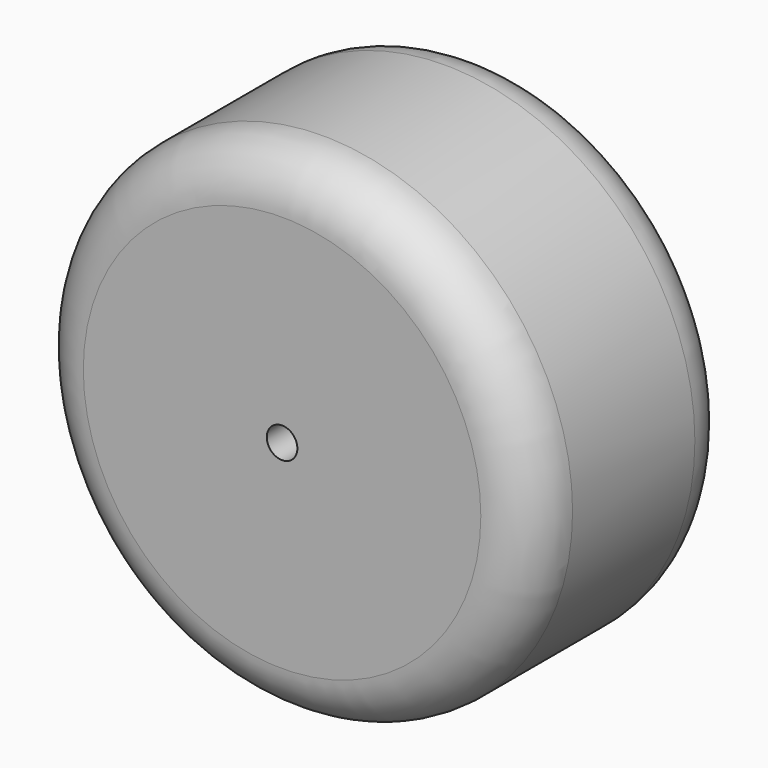
from build123d import *

# Parameters (mm, degrees)
F0_R     = 49
F1_DEPTH = 50
F2_R     = 10
F4_R     = 25.5
F4_R_2   = 6.5
F5_DEPTH = 12
F6_DEPTH = 15
F7_R     = 11.99999
F4_R_3   = 3
F8_DEPTH = 50.001


# Not quite as in the source:
# - a fillet or chamfer is up to 0.001 mm smaller than in the source, because OpenCascade refuses the exact size


with BuildPart() as f1:
    # F0 (on Front) → F1 (new body)
    with BuildSketch(Plane.XZ):
        Circle(F0_R)
    extrude(amount=F1_DEPTH)

    # F2
    f2_edges = [f1.edges().sort_by_distance(p)[0] for p in [
        (-49, -50, 0),
        (-49, 0, 0),
    ]]
    fillet(f2_edges, radius=F2_R)

    # F4 (on Front) → F5 (cut)
    with BuildSketch(Plane.XZ):
        Circle(F4_R)
        Circle(F4_R_2, mode=Mode.SUBTRACT)
    extrude(amount=F5_DEPTH, mode=Mode.SUBTRACT)

    # F6 (cut): a face of the model
    f6_faces = [f1.faces().sort_by_distance(p)[0] for p in [
        (0, 0, 0),
    ]]
    extrude(f6_faces, amount=-F6_DEPTH, mode=Mode.SUBTRACT)

    # F7 (radius 12 in the source; OpenCascade refuses exactly that, so slightly less here)
    f7_edges = [f1.edges().sort_by_distance(p)[0] for p in [
        (-25.5, -12, 0),
    ]]
    fillet(f7_edges, radius=F7_R)

    # F4 (on Front) → F8 (cut, through all)
    with BuildSketch(Plane.XZ):
        Circle(F4_R_3)
    extrude(amount=F8_DEPTH, mode=Mode.SUBTRACT)


solid = f1.part
